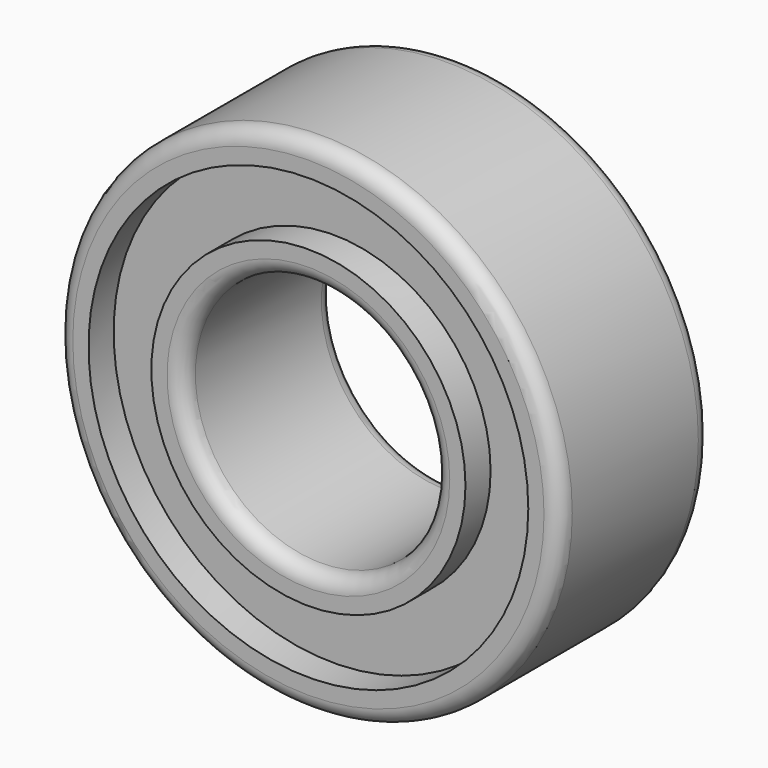
from build123d import *

# Parameters (mm, degrees)
F0_R     = 6.35
F0_R_2   = 3.175
F1_DEPTH = 2.3876
F2_R     = 5.55625
F2_R_2   = 3.96875
F3_DEPTH = 0.79375
F4_R     = 0.396875


# Not quite as in the source:
# - a pattern or mirror of a feature is missing from the dataset's text; its kind, count and spacing are read off the source's solid


with BuildPart() as f1:
    # F0 (on Front) → F1 (new body, symmetric)
    with BuildSketch(Plane.XZ):
        Circle(F0_R)
        Circle(F0_R_2, mode=Mode.SUBTRACT)
    extrude(amount=F1_DEPTH, both=True)

    # F2 (on face) → F3 (cut)
    with BuildSketch(Plane.XZ.offset(2.3876)):
        Circle(F2_R)
        Circle(F2_R_2, mode=Mode.SUBTRACT)
    f3 = extrude(amount=-F3_DEPTH, mode=Mode.SUBTRACT)

    # F3_copies: F3 across plane
    add(f3.mirror(Plane.ZX), mode=Mode.SUBTRACT)

    # F4
    f4_edges = [f1.edges().sort_by_distance(p)[0] for p in [
        (-3.175, -2.3876, 0),
        (3.175, 0, 0),
        (-3.175, 2.3876, 0),
        (-6.35, 2.3876, 0),
        (6.35, 0, 0),
        (-6.35, -2.3876, 0),
    ]]
    fillet(f4_edges, radius=F4_R)


solid = f1.part
